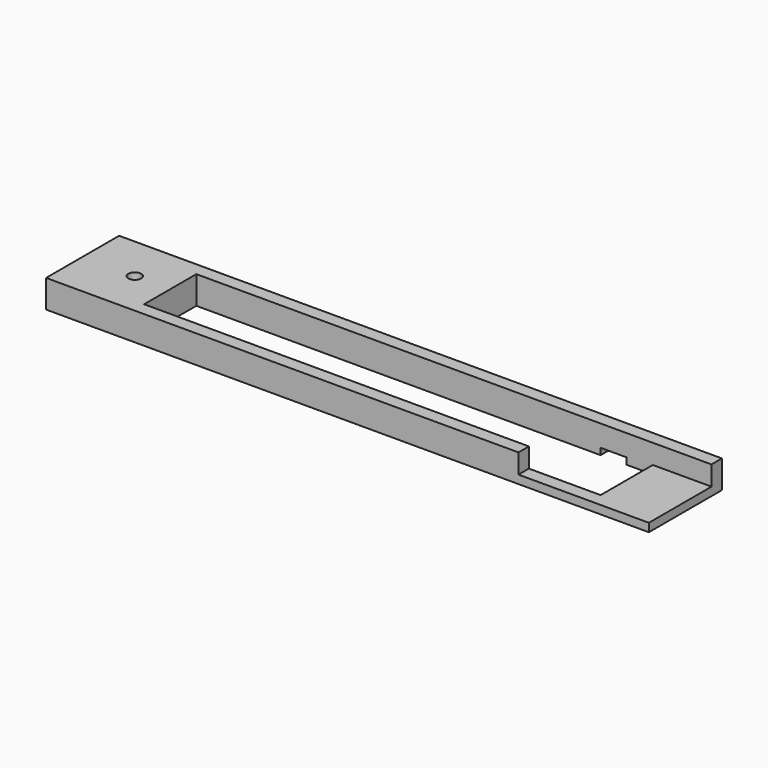
from build123d import *

# Parameters (mm, degrees)
F0_W      = 117.3988
F0_H      = 17.78
F1_DEPTH  = 5.4356
F2_W      = 88.9
F2_H      = 12.7
F3_DEPTH  = 25.4
F4_W      = 11.43
F4_H      = 12.7
F5_DEPTH  = 3.81
F7_DEPTH  = 169
F8_R      = 1.24968
F9_DEPTH  = 5.4356
F10_W     = 5.08
F10_H     = 2.54
F11_DEPTH = 1.27


# Not quite as in the source:
# - an extrude ends at something that could not be found from the text; its depth is read off the source's solid


with BuildPart() as f1:
    # F0 (on Top) → F1 (new body)
    with BuildSketch(Plane.XY):
        with Locations((58.6994, 8.89)):
            Rectangle(F0_W, F0_H)
    extrude(amount=F1_DEPTH)

    # F2 (on face) → F3 (cut)
    with BuildSketch(Plane.XY.offset(5.4356)):
        with Locations((61.5188, 8.89)):
            Rectangle(F2_W, F2_H)
    extrude(amount=-F3_DEPTH, mode=Mode.SUBTRACT)

    # F4 (on face) → F5 (cut)
    with BuildSketch(Plane.XY.offset(5.4356)):
        with Locations((111.6838, 8.89)):
            Rectangle(F4_W, F4_H)
    extrude(amount=-F5_DEPTH, mode=Mode.SUBTRACT)

    # F6 (on face) → F7 (cut, through all)
    with BuildSketch(Plane.XY.offset(1.6256)):
        Polygon((105.9688, 2.54), (105.9688, 15.24), (91.9988, 15.24), (91.9988, 0), (117.3988, 0), (117.3988, 2.54), align=None)
    extrude(amount=F7_DEPTH, mode=Mode.SUBTRACT)

    # F8 (on face) → F9 (cut, through all)
    with BuildSketch(Plane.XY.offset(5.4356)):
        with Locations((10.16, 8.89)):
            Circle(F8_R)
    extrude(amount=-F9_DEPTH, mode=Mode.SUBTRACT)

    # F10 (on face) → F11 (cut)
    with BuildSketch(Plane(origin=(0, 0, 0), x_dir=(1, 0, 0), z_dir=(0, 0, -1))):
        with Locations((98.3488, -16.51)):
            Rectangle(F10_W, F10_H)
        Polygon((95.8088, -15.24), (100.8888, -15.24), (105.9688, -15.24), (105.9688, -2.54), (17.0688, -2.54), (17.0688, -15.24), align=None)
    extrude(amount=-F11_DEPTH, mode=Mode.SUBTRACT)


solid = f1.part
